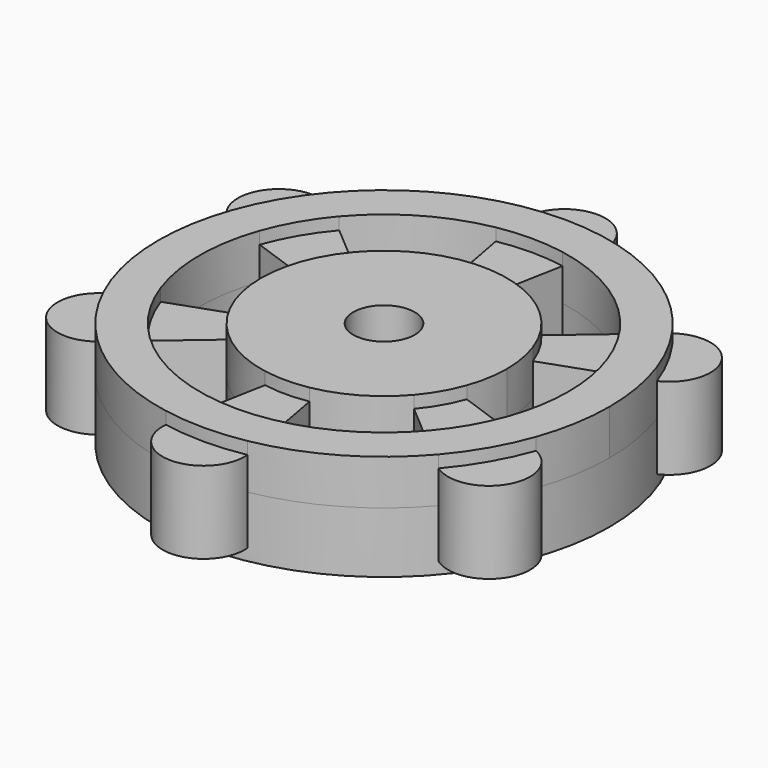
from build123d import *

# Parameters (mm, degrees)
F0_R          = 17.4625
F0_R_2        = 14.2875
F1_DEPTH      = 4.7085
F0_R_3        = 9.525
F3_DEPTH      = 2.54
F3_DEPTH_BACK = 3.81
F2_R          = 2.38125
F4_DEPTH      = 3.4925


# Not quite as in the source:
# - a feature names something its author has since deleted; it is built from what else it names


with BuildPart() as f1:
    # F0 (on Top) → F1 (new body)
    with BuildSketch(Plane.XY):
        Circle(F0_R)
        Circle(F0_R_2, mode=Mode.SUBTRACT)
    extrude(amount=F1_DEPTH)



with BuildPart() as f1b:
    # F0 (on Top) → F1, piece 2 (new body)
    with BuildSketch(Plane.XY):
        Circle(F0_R_3)
        Polygon((0, -5.715), (-4.9493351826, -2.8575), (-4.9493351826, 2.8575), (0, 5.715), (4.9493351826, 2.8575), (4.9493351826, -2.8575), align=None, mode=Mode.SUBTRACT)
    extrude(amount=F1_DEPTH)


with BuildPart() as f3:
    # F2 (on face) → F3 (new body, two sides)
    with BuildSketch(Plane.XY.offset(4.7085)) as f3_sk:
        with BuildLine():
            ThreePointArc((3.1618529456, -17.1738636364), (0, -17.4625), (-3.1618529456, -17.1738636364))
            ThreePointArc((-3.1618529456, -17.1738636364), (0, -20.6375), (3.1618529456, -17.1738636364))
        make_face()
    extrude(amount=F3_DEPTH)
    extrude(f3_sk.sketch, amount=-F3_DEPTH_BACK)


with BuildPart() as f3b:
    # F2 (on face) → F3, piece 2 (new body, two sides)
    with BuildSketch(Plane.XY.offset(4.7085)) as f3_2_sk:
        with BuildLine():
            ThreePointArc((-16.453928663, -5.8486868443), (-17.8725992706, -10.31875), (-13.2920757174, -11.3251767921))
            ThreePointArc((-13.2920757174, -11.3251767921), (-15.1229686136, -8.73125), (-16.453928663, -5.8486868443))
        make_face()
    extrude(amount=F3_DEPTH)
    extrude(f3_2_sk.sketch, amount=-F3_DEPTH_BACK)


with BuildPart() as f3c:
    # F2 (on face) → F3, piece 3 (new body, two sides)
    with BuildSketch(Plane.XY.offset(4.7085)) as f3_3_sk:
        with BuildLine():
            ThreePointArc((-13.2920757174, 11.3251767921), (-17.8725992706, 10.31875), (-16.453928663, 5.8486868443))
            ThreePointArc((-16.453928663, 5.8486868443), (-15.1229686136, 8.73125), (-13.2920757174, 11.3251767921))
        make_face()
    extrude(amount=F3_DEPTH)
    extrude(f3_3_sk.sketch, amount=-F3_DEPTH_BACK)


with BuildPart() as f3d:
    # F2 (on face) → F3, piece 4 (new body, two sides)
    with BuildSketch(Plane.XY.offset(4.7085)) as f3_4_sk:
        with BuildLine():
            ThreePointArc((3.1618529456, 17.1738636364), (0, 20.6375), (-3.1618529456, 17.1738636364))
            ThreePointArc((-3.1618529456, 17.1738636364), (0, 17.4625), (3.1618529456, 17.1738636364))
        make_face()
    extrude(amount=F3_DEPTH)
    extrude(f3_4_sk.sketch, amount=-F3_DEPTH_BACK)


with BuildPart() as f3e:
    # F2 (on face) → F3, piece 5 (new body, two sides)
    with BuildSketch(Plane.XY.offset(4.7085)) as f3_5_sk:
        with BuildLine():
            ThreePointArc((13.2920757174, 11.3251767921), (15.1229686136, 8.73125), (16.453928663, 5.8486868443))
            ThreePointArc((16.453928663, 5.8486868443), (17.8725992706, 10.31875), (13.2920757174, 11.3251767921))
        make_face()
    extrude(amount=F3_DEPTH)
    extrude(f3_5_sk.sketch, amount=-F3_DEPTH_BACK)


with BuildPart() as f3f:
    # F2 (on face) → F3, piece 6 (new body, two sides)
    with BuildSketch(Plane.XY.offset(4.7085)) as f3_6_sk:
        with BuildLine():
            ThreePointArc((16.453928663, -5.8486868443), (15.1229686136, -8.73125), (13.2920757174, -11.3251767921))
            ThreePointArc((13.2920757174, -11.3251767921), (17.8725992706, -10.31875), (16.453928663, -5.8486868443))
        make_face()
    extrude(amount=F3_DEPTH)
    extrude(f3_6_sk.sketch, amount=-F3_DEPTH_BACK)


with BuildPart() as f3g:
    # F2 (on face) → F3, piece 7 (new body, two sides)
    with BuildSketch(Plane.XY.offset(4.7085)) as f3_7_sk:
        with BuildLine():
            ThreePointArc((8.9711821608, -3.2005492712), (8.248891971, -4.7625), (7.2573480553, -6.1689970177))
            Line((7.2573480553, -6.1689970177), (10.8781860674, -9.2627060912))
            ThreePointArc((10.8781860674, -9.2627060912), (12.3733379566, -7.14375), (13.4608318165, -4.7894324359))
            Line((13.4608318165, -4.7894324359), (8.9711821608, -3.2005492712))
        make_face()
    extrude(amount=F3_DEPTH)
    extrude(f3_7_sk.sketch, amount=-F3_DEPTH_BACK)


with BuildPart() as f3h:
    # F2 (on face) → F3, piece 8 (new body, two sides)
    with BuildSketch(Plane.XY.offset(4.7085)) as f3_8_sk:
        with BuildLine():
            ThreePointArc((7.2573480553, 6.1689970177), (8.248891971, 4.7625), (8.9711821608, 3.2005492712))
            Line((8.9711821608, 3.2005492712), (13.4608318165, 4.7894324359))
            ThreePointArc((13.4608318165, 4.7894324359), (12.3733379566, 7.14375), (10.8781860674, 9.2627060912))
            Line((10.8781860674, 9.2627060912), (7.2573480553, 6.1689970177))
        make_face()
    extrude(amount=F3_DEPTH)
    extrude(f3_8_sk.sketch, amount=-F3_DEPTH_BACK)


with BuildPart() as f3i:
    # F2 (on face) → F3, piece 9 (new body, two sides)
    with BuildSketch(Plane.XY.offset(4.7085)) as f3_9_sk:
        with BuildLine():
            Line((-2.5826457491, 14.0521385271), (-1.7138341055, 9.3695462888))
            ThreePointArc((-1.7138341055, 9.3695462888), (0, 9.525), (1.7138341055, 9.3695462888))
            Line((1.7138341055, 9.3695462888), (2.5826457491, 14.0521385271))
            ThreePointArc((2.5826457491, 14.0521385271), (0, 14.2875), (-2.5826457491, 14.0521385271))
        make_face()
    extrude(amount=F3_DEPTH)
    extrude(f3_9_sk.sketch, amount=-F3_DEPTH_BACK)


with BuildPart() as f3j:
    # F2 (on face) → F3, piece 10 (new body, two sides)
    with BuildSketch(Plane.XY.offset(4.7085)) as f3_10_sk:
        with BuildLine():
            Line((-10.8781860674, -9.2627060912), (-7.2573480553, -6.1689970177))
            ThreePointArc((-7.2573480553, -6.1689970177), (-8.248891971, -4.7625), (-8.9711821608, -3.2005492712))
            Line((-8.9711821608, -3.2005492712), (-13.4608318165, -4.7894324359))
            ThreePointArc((-13.4608318165, -4.7894324359), (-12.3733379566, -7.14375), (-10.8781860674, -9.2627060912))
        make_face()
    extrude(amount=F3_DEPTH)
    extrude(f3_10_sk.sketch, amount=-F3_DEPTH_BACK)


with BuildPart() as f3k:
    # F2 (on face) → F3, piece 11 (new body, two sides)
    with BuildSketch(Plane.XY.offset(4.7085)) as f3_11_sk:
        with BuildLine():
            ThreePointArc((1.7246470612, -9.3675619835), (0.0054967599, -9.5249984139), (-1.7138341055, -9.3695462888))
            Line((-1.7138341055, -9.3695462888), (-2.5826457491, -14.0521385271))
            ThreePointArc((-2.5826457491, -14.0521385271), (0.0021987023, -14.2874998308), (2.5869705919, -14.0513429752))
            Line((2.5869705919, -14.0513429752), (1.7246470612, -9.3675619835))
        make_face()
    extrude(amount=F3_DEPTH)
    extrude(f3_11_sk.sketch, amount=-F3_DEPTH_BACK)


with BuildPart() as f3l:
    # F2 (on face) → F3, piece 12 (new body, two sides)
    with BuildSketch(Plane.XY.offset(4.7085)) as f3_12_sk:
        with BuildLine():
            Line((-13.4608318165, 4.7894324359), (-8.9711821608, 3.2005492712))
            ThreePointArc((-8.9711821608, 3.2005492712), (-8.248891971, 4.7625), (-7.2573480553, 6.1689970177))
            Line((-7.2573480553, 6.1689970177), (-10.8781860674, 9.2627060912))
            ThreePointArc((-10.8781860674, 9.2627060912), (-12.3733379566, 7.14375), (-13.4608318165, 4.7894324359))
        make_face()
    extrude(amount=F3_DEPTH)
    extrude(f3_12_sk.sketch, amount=-F3_DEPTH_BACK)


with BuildPart() as f1_1:
    add(f1.part)

    add(f1b.part)  # F4 merges F1b

    add(f3.part)  # F4 merges F3

    add(f3b.part)  # F4 merges F3b

    add(f3c.part)  # F4 merges F3c

    add(f3d.part)  # F4 merges F3d

    add(f3e.part)  # F4 merges F3e

    add(f3f.part)  # F4 merges F3f

    add(f3g.part)  # F4 merges F3g

    add(f3h.part)  # F4 merges F3h

    add(f3i.part)  # F4 merges F3i

    add(f3j.part)  # F4 merges F3j

    add(f3k.part)  # F4 merges F3k

    add(f3l.part)  # F4 merges F3l
    # F2 (on face) → F4 (join)
    with BuildSketch(Plane.XY.offset(4.7085)):
        with BuildLine():
            ThreePointArc((-13.2920757174, -11.3251767921), (-8.73125, -15.1229686136), (-3.1618529456, -17.1738636364))
            ThreePointArc((-3.1618529456, -17.1738636364), (0, -17.4625), (3.1618529456, -17.1738636364))
            ThreePointArc((3.1618529456, -17.1738636364), (8.73125, -15.1229686136), (13.2920757174, -11.3251767921))
            ThreePointArc((13.2920757174, -11.3251767921), (15.1229686136, -8.73125), (16.453928663, -5.8486868443))
            ThreePointArc((16.453928663, -5.8486868443), (17.208510039, -2.9675054315), (17.4625, 0))
            ThreePointArc((17.4625, 0), (17.208510039, 2.9675054315), (16.453928663, 5.8486868443))
            ThreePointArc((16.453928663, 5.8486868443), (15.1229686136, 8.73125), (13.2920757174, 11.3251767921))
            ThreePointArc((13.2920757174, 11.3251767921), (8.73125, 15.1229686136), (3.1618529456, 17.1738636364))
            ThreePointArc((3.1618529456, 17.1738636364), (0, 17.4625), (-3.1618529456, 17.1738636364))
            ThreePointArc((-3.1618529456, 17.1738636364), (-8.73125, 15.1229686136), (-13.2920757174, 11.3251767921))
            ThreePointArc((-13.2920757174, 11.3251767921), (-15.1229686136, 8.73125), (-16.453928663, 5.8486868443))
            ThreePointArc((-16.453928663, 5.8486868443), (-17.4625, 0), (-16.453928663, -5.8486868443))
            ThreePointArc((-16.453928663, -5.8486868443), (-15.1229686136, -8.73125), (-13.2920757174, -11.3251767921))
        make_face()
        with BuildLine():
            ThreePointArc((2.5869705919, -14.0513429752), (0.0021987023, -14.2874998308), (-2.5826457491, -14.0521385271))
            ThreePointArc((-2.5826457491, -14.0521385271), (-7.14375, -12.3733379566), (-10.8781860674, -9.2627060912))
            ThreePointArc((-10.8781860674, -9.2627060912), (-12.3733379566, -7.14375), (-13.4608318165, -4.7894324359))
            ThreePointArc((-13.4608318165, -4.7894324359), (-14.2875, 0), (-13.4608318165, 4.7894324359))
            ThreePointArc((-13.4608318165, 4.7894324359), (-12.3733379566, 7.14375), (-10.8781860674, 9.2627060912))
            ThreePointArc((-10.8781860674, 9.2627060912), (-7.14375, 12.3733379566), (-2.5826457491, 14.0521385271))
            ThreePointArc((-2.5826457491, 14.0521385271), (0, 14.2875), (2.5826457491, 14.0521385271))
            ThreePointArc((2.5826457491, 14.0521385271), (7.14375, 12.3733379566), (10.8781860674, 9.2627060912))
            ThreePointArc((10.8781860674, 9.2627060912), (12.3733379566, 7.14375), (13.4608318165, 4.7894324359))
            ThreePointArc((13.4608318165, 4.7894324359), (14.0793162268, 2.4301256831), (14.2875, 0))
            ThreePointArc((14.2875, 0), (14.0793162268, -2.4301256831), (13.4608318165, -4.7894324359))
            ThreePointArc((13.4608318165, -4.7894324359), (12.3733379566, -7.14375), (10.8781860674, -9.2627060912))
            ThreePointArc((10.8781860674, -9.2627060912), (7.1456540475, -12.3722384589), (2.5869705919, -14.0513429752))
        make_face(mode=Mode.SUBTRACT)
        with BuildLine():
            ThreePointArc((-7.2573480553, -6.1689970177), (-4.7625, -8.248891971), (-1.7138341055, -9.3695462888))
            ThreePointArc((-1.7138341055, -9.3695462888), (0.0054967599, -9.5249984139), (1.7246470612, -9.3675619835))
            ThreePointArc((1.7246470612, -9.3675619835), (4.7672595407, -8.2461422175), (7.2573480553, -6.1689970177))
            ThreePointArc((7.2573480553, -6.1689970177), (8.248891971, -4.7625), (8.9711821608, -3.2005492712))
            ThreePointArc((8.9711821608, -3.2005492712), (9.3855243615, -1.624055867), (9.525, 0))
            ThreePointArc((9.525, 0), (9.3855243615, 1.624055867), (8.9711821608, 3.2005492712))
            ThreePointArc((8.9711821608, 3.2005492712), (8.248891971, 4.7625), (7.2573480553, 6.1689970177))
            ThreePointArc((7.2573480553, 6.1689970177), (4.7625, 8.248891971), (1.7138341055, 9.3695462888))
            ThreePointArc((1.7138341055, 9.3695462888), (0, 9.525), (-1.7138341055, 9.3695462888))
            ThreePointArc((-1.7138341055, 9.3695462888), (-4.7625, 8.248891971), (-7.2573480553, 6.1689970177))
            ThreePointArc((-7.2573480553, 6.1689970177), (-8.248891971, 4.7625), (-8.9711821608, 3.2005492712))
            ThreePointArc((-8.9711821608, 3.2005492712), (-9.525, 0), (-8.9711821608, -3.2005492712))
            ThreePointArc((-8.9711821608, -3.2005492712), (-8.248891971, -4.7625), (-7.2573480553, -6.1689970177))
        make_face()
        Polygon((4.9493351826, 2.8575), (4.9493351826, -2.8575), (0, -5.715), (-4.9493351826, -2.8575), (-4.9493351826, 2.8575), (0, 5.715), align=None, mode=Mode.SUBTRACT)
        Polygon((0, -5.715), (4.9493351826, -2.8575), (4.9493351826, 2.8575), (0, 5.715), (-4.9493351826, 2.8575), (-4.9493351826, -2.8575), align=None)
        Circle(F2_R, mode=Mode.SUBTRACT)
    extrude(amount=F4_DEPTH)


solid = f1_1.part
